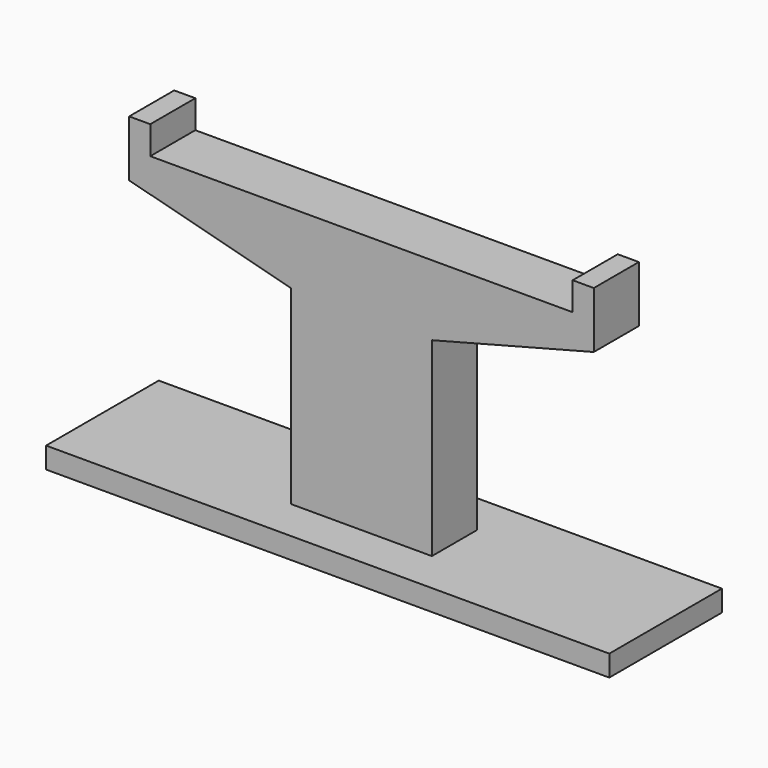
from build123d import *

# Parameters (mm, degrees)
F4_W      = 40
F4_H      = 10
F4_W_2    = 10
F4_H_2    = 4
F5_DEPTH  = 1.5
F6_DEPTH  = 20
F7_W      = 33
F7_H      = 4
F8_DEPTH  = 5
F9_SIZE2  = 2.99999
F9_SIZE   = 11.49999
F10_SIZE2 = 11.49999
F10_SIZE  = 2.99999
F11_W     = 1.5
F11_H     = 4
F12_DEPTH = 2


# Not quite as in the source:
# - a fillet or chamfer is up to 0.001 mm smaller than in the source, because OpenCascade refuses the exact size


with BuildPart() as f5:
    # F4 (on Top) → F5 (new body)
    with BuildSketch(Plane.XY):
        Rectangle(F4_W, F4_H)
        Rectangle(F4_W_2, F4_H_2, mode=Mode.SUBTRACT)
    extrude(amount=F5_DEPTH)

    # F4 (on Top) → F6 (join)
    with BuildSketch(Plane.XY):
        Rectangle(F4_W_2, F4_H_2)
    extrude(amount=F6_DEPTH)

    # F7 (on face) → F8 (join)
    with BuildSketch(Plane.XY.offset(20)):
        Rectangle(F7_W, F7_H)
    extrude(amount=-F8_DEPTH)

    # F9 (size 11.5 and 3 in the source; OpenCascade refuses exactly that, so slightly less here)
    f9_edges = [f5.edges().sort_by_distance(p)[0] for p in [
        (16.5, 0, 15),
    ]]
    f9_side = f5.faces().sort_by_distance((10.75, 0, 15))[0]
    chamfer(f9_edges, length=F9_SIZE, length2=F9_SIZE2, reference=f9_side)

    # F10 (size 3 and 11.5 in the source; OpenCascade refuses exactly that, so slightly less here)
    f10_edges = [f5.edges().sort_by_distance(p)[0] for p in [
        (-16.5, 0, 15),
    ]]
    f10_side = f5.faces().sort_by_distance((-16.5, 0, 17.5))[0]
    chamfer(f10_edges, length=F10_SIZE, length2=F10_SIZE2, reference=f10_side)

    # F11 (on face) → F12 (join)
    with BuildSketch(Plane.XY.offset(20)):
        with Locations((15.75, 0)):
            Rectangle(F11_W, F11_H)
        with Locations((-15.75, 0)):
            Rectangle(F11_W, F11_H)
    extrude(amount=F12_DEPTH)


solid = f5.part
